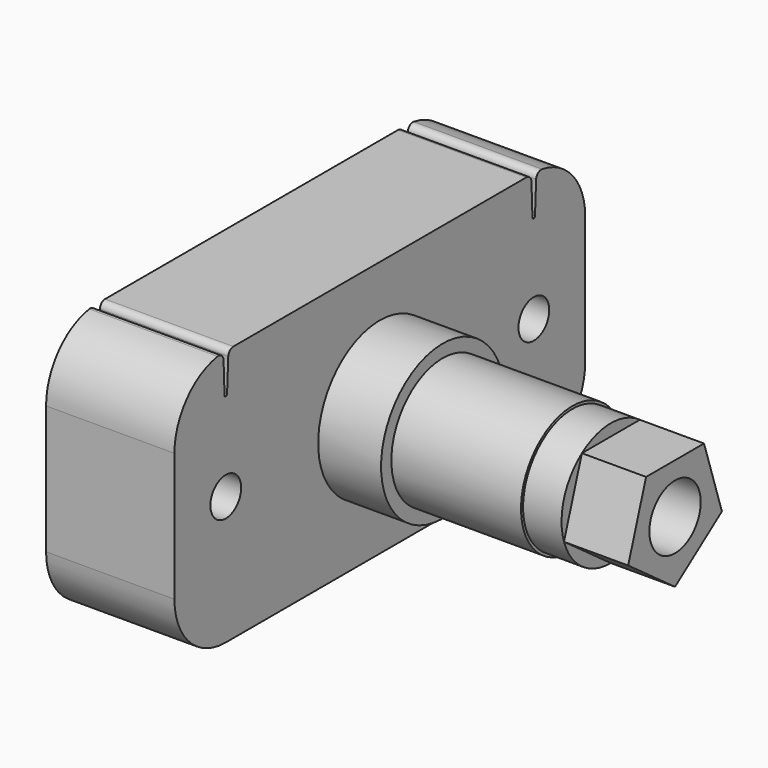
from build123d import *

# Parameters (mm, degrees)
F0_R          = 5
F1_DEPTH      = 25
F2_R          = 4.8
F3_DEPTH      = 3
F5_DEPTH      = 5
F5_DEPTH_BACK = 23
F6_W          = 40
F6_H          = 20
F6_R          = 1.5
F7_DEPTH      = 10
F9_DEPTH      = 10
F10_T1_DEPTH  = 34.9696394511
F10_T3_DEPTH  = 35
F10_T5_DEPTH  = 34.9715357564
F11_R         = 0.5
F12_R         = 6
F13_DEPTH     = 4.9
F14_R         = 2.5
F15_DEPTH     = 65


# Not quite as in the source:
# - a fillet or chamfer that OpenCascade refuses, or shapes differently, is made with other operations: its cross-section is extruded or revolved along the edge and cut away or added
# - a feature names something its author has since deleted; it is built from what else it names


with BuildPart() as f1:
    # F0 (on Right) → F1 (new body)
    with BuildSketch(Plane.YZ):
        Circle(F0_R)
    extrude(amount=-F1_DEPTH)

    # F2 (on face) → F3 (join)
    with BuildSketch(Plane.YZ):
        Circle(F2_R)
    extrude(amount=F3_DEPTH)

    # F4 (on face) → F5 (join, two sides)
    with BuildSketch(Plane.YZ.offset(3)) as f5_sk:
        Polygon((-4.5650712782, -1.483281573), (0, -4.8), (4.5650712782, -1.483281573), (2.821369211, 3.883281573), (-2.821369211, 3.883281573), align=None)
    extrude(amount=F5_DEPTH)
    extrude(f5_sk.sketch, amount=-F5_DEPTH_BACK)

    # F6 (on face) → F7 (join)
    with BuildSketch(Plane(origin=(-25, 0, 0), x_dir=(0, -1, 0), z_dir=(-1, 0, 0))):
        Rectangle(F6_W, F6_H)
        with Locations((-15, 0)):
            Circle(F6_R, mode=Mode.SUBTRACT)
        with BuildLine():
            ThreePointArc((13.5, 0), (15, 1.5), (16.5, 0))
            ThreePointArc((16.5, 0), (15, -1.5), (13.5, 0))
        make_face(mode=Mode.SUBTRACT)
    extrude(amount=-F7_DEPTH)

    # F8 (on face) → F9 (cut)
    with BuildSketch(Plane(origin=(-25, 0, 0), x_dir=(0, -1, 0), z_dir=(-1, 0, 0))):
        with BuildLine():
            Line((15.0452693954, 10), (14.9885289893, 10))
            Line((14.9885289893, 10), (14.7385289893, 10))
            Line((14.7385289893, 10), (14.8751285557, 6.9943249556))
            ThreePointArc((14.8751285557, 6.9943249556), (15.0159151334, 6.8760173486), (15.1222554927, 7.0260482732))
            Line((15.1222554927, 7.0260482732), (15.2385289893, 10))
            Line((15.2385289893, 10), (15.0452693954, 10))
        make_face()
        with BuildLine():
            Line((-14.9398591969, 10.0056750444), (-14.9965996031, 10.0056750444))
            Line((-14.9965996031, 10.0056750444), (-15.2465996031, 10.0056750444))
            Line((-15.2465996031, 10.0056750444), (-15.1100000367, 7))
            ThreePointArc((-15.1100000367, 7), (-14.9692134589, 6.881692393), (-14.8628730997, 7.0317233176))
            Line((-14.8628730997, 7.0317233176), (-14.7465996031, 10.0056750444))
            Line((-14.7465996031, 10.0056750444), (-14.9398591969, 10.0056750444))
        make_face()
    extrude(amount=-F9_DEPTH, mode=Mode.SUBTRACT)

    # F10: fillet of radius 5 on 4 edges, made by hand

    # F10_s2 → F10_t1 (cut)
    with BuildSketch(Plane.YZ.offset(-37.4848197255)):
        with BuildLine():
            ThreePointArc((20, 5.0060721098), (18.6215817291, 8.4534110516), (15.2463416881, 10))
            Line((15.2463416881, 10), (20, 10))
            Line((20, 10), (20, 5.0060721098))
        make_face()
    extrude(amount=F10_T1_DEPTH, mode=Mode.SUBTRACT)

    # F10_s4 → F10_t3 (cut)
    with BuildSketch(Plane.YZ.offset(-37.5)):
        with BuildLine():
            ThreePointArc((15, -10), (18.5355339059, -8.5355339059), (20, -5))
            Line((20, -5), (20, -10))
            Line((20, -10), (15, -10))
        make_face()
        with BuildLine():
            ThreePointArc((-20, -5), (-18.5355339059, -8.5355339059), (-15, -10))
            Line((-15, -10), (-20, -10))
            Line((-20, -10), (-20, -5))
        make_face()
    extrude(amount=F10_T3_DEPTH, mode=Mode.SUBTRACT)

    # F10_s6 → F10_t5 (cut)
    with BuildSketch(Plane.YZ.offset(-37.4857678782)):
        with BuildLine():
            ThreePointArc((-20, 5.0056928487), (-18.6188841475, 8.4558635006), (-15.2385289893, 10))
            Line((-15.2385289893, 10), (-20, 10))
            Line((-20, 10), (-20, 5.0056928487))
        make_face()
    extrude(amount=F10_T5_DEPTH, mode=Mode.SUBTRACT)

    # F11
    f11_edges = [f1.edges().sort_by_distance(p)[0] for p in [
        (-20, -14.738529, 10),
        (-20, 14.746821, 10),
        (-20, 15.246342, 10),
        (-20, -15.238529, 10),
    ]]
    fillet(f11_edges, radius=F11_R)

    # F12 (on face) → F13 (join)
    with BuildSketch(Plane.YZ.offset(-15)):
        Circle(F12_R)
    extrude(amount=F13_DEPTH)

    # F14 (on face) → F15 (cut)
    with BuildSketch(Plane.YZ.offset(8)):
        Circle(F14_R)
    extrude(amount=-F15_DEPTH, mode=Mode.SUBTRACT)


solid = f1.part
